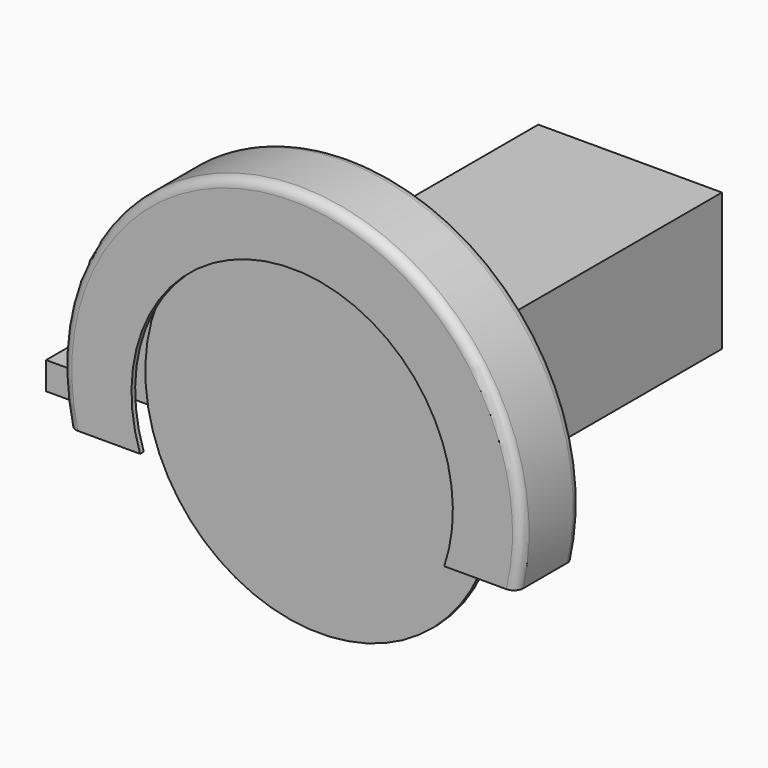
from build123d import *

# Parameters (mm, degrees)
F1_DEPTH  = 20
F2_T      = -2.5
F3_START  = -17.5
F3_DEPTH  = 2.5
F4_START  = -17.5
F0_W      = 100
F0_H      = 75
F4_DEPTH  = 192.5
F5_R      = 5
F6_DEPTH  = 1.2
F7_W      = 15
F7_H      = 15
F8_DEPTH  = 100
F9_W      = 15
F9_H      = 15
F10_DEPTH = 20


with BuildPart() as f1:
    # F0 (on Front) → F1 (new body, symmetric)
    with BuildSketch(Plane.XZ):
        with BuildLine():
            ThreePointArc((-93.7288880384, -32.7305903801), (-17.3139573127, 89.4389150959), (91.973567456, -4.4805537909))
            ThreePointArc((91.973567456, -4.4805537909), (90.8930363428, -18.7680785596), (87.6760229504, -32.7305903801))
            Line((87.6760229504, -32.7305903801), (118.739471685, -32.7305903801))
            ThreePointArc((118.739471685, -32.7305903801), (-3.026432544, 120.5194462091), (-124.792336773, -32.7305903801))
            Line((-124.792336773, -32.7305903801), (-93.7288880384, -32.7305903801))
        make_face()
        with BuildLine():
            ThreePointArc((87.6760229504, -32.7305903801), (90.8930363428, -18.7680785596), (91.973567456, -4.4805537909))
            ThreePointArc((91.973567456, -4.4805537909), (-17.3139573127, 89.4389150959), (-93.7288880384, -32.7305903801))
            Line((-93.7288880384, -32.7305903801), (-85.8405945739, -32.7305903801))
            ThreePointArc((-85.8405945739, -32.7305903801), (-3.026432544, 83.0194462091), (79.7877294859, -32.7305903801))
            Line((79.7877294859, -32.7305903801), (87.6760229504, -32.7305903801))
        make_face()
    extrude(amount=F1_DEPTH, both=True)

    # F2
    f2_openings = [f1.faces().sort_by_distance(p)[0] for p in [
        (-3.026433, 0, 83.019446),
        (99.263601, 0, -32.73059),
        (-105.316466, 0, -32.73059),
    ]]
    offset(amount=F2_T, openings=f2_openings)

    # F0 (on Front) → F3 (join)
    with BuildSketch(Plane.XZ.offset(F3_START)):
        with BuildLine():
            ThreePointArc((79.7877294859, -32.7305903801), (-3.026432544, 83.0194462091), (-85.8405945739, -32.7305903801))
            Line((-85.8405945739, -32.7305903801), (-53.026432544, -32.7305903801))
            Line((-53.026432544, -32.7305903801), (-53.026432544, 42.2694096199))
            Line((-53.026432544, 42.2694096199), (46.973567456, 42.2694096199))
            Line((46.973567456, 42.2694096199), (46.973567456, -32.7305903801))
            Line((46.973567456, -32.7305903801), (79.7877294859, -32.7305903801))
        make_face()
    extrude(amount=-F3_DEPTH)

    # F0 (on Front) → F4 (join)
    with BuildSketch(Plane.XZ.offset(F4_START)):
        with Locations((-3.026432544, 4.7694096199)):
            Rectangle(F0_W, F0_H)
    extrude(amount=-F4_DEPTH)

    # F5
    f5_edges = [f1.edges().sort_by_distance(p)[0] for p in [
        (-3.026433, -20, 120.519446),
        (-3.026433, 20, 120.519446),
    ]]
    fillet(f5_edges, radius=F5_R)

    # F7 (on face) → F8 (join)
    with BuildSketch(Plane(origin=(-53.026432544, 0, 0), x_dir=(0, -1, 0), z_dir=(-1, 0, 0))):
        with Locations((-27.5, -25.2305903801)):
            Rectangle(F7_W, F7_H)
    extrude(amount=F8_DEPTH)


with BuildPart() as f6:
    # F0 (on Front) → F6 (new body, symmetric)
    with BuildSketch(Plane.XZ):
        with BuildLine():
            ThreePointArc((87.6760229504, -32.7305903801), (90.8930363428, -18.7680785596), (91.973567456, -4.4805537909))
            ThreePointArc((91.973567456, -4.4805537909), (-17.3139573127, 89.4389150959), (-93.7288880384, -32.7305903801))
            Line((-93.7288880384, -32.7305903801), (-85.8405945739, -32.7305903801))
            ThreePointArc((-85.8405945739, -32.7305903801), (-3.026432544, 83.0194462091), (79.7877294859, -32.7305903801))
            Line((79.7877294859, -32.7305903801), (87.6760229504, -32.7305903801))
        make_face()
        with BuildLine():
            ThreePointArc((79.7877294859, -32.7305903801), (-3.026432544, 83.0194462091), (-85.8405945739, -32.7305903801))
            Line((-85.8405945739, -32.7305903801), (-53.026432544, -32.7305903801))
            Line((-53.026432544, -32.7305903801), (-53.026432544, 42.2694096199))
            Line((-53.026432544, 42.2694096199), (46.973567456, 42.2694096199))
            Line((46.973567456, 42.2694096199), (46.973567456, -32.7305903801))
            Line((46.973567456, -32.7305903801), (79.7877294859, -32.7305903801))
        make_face()
        with Locations((-3.026432544, 4.7694096199)):
            Rectangle(F0_W, F0_H)
        with BuildLine():
            Line((-85.8405945739, -32.7305903801), (-93.7288880384, -32.7305903801))
            ThreePointArc((-93.7288880384, -32.7305903801), (-3.026432544, -99.4805537909), (87.6760229504, -32.7305903801))
            Line((87.6760229504, -32.7305903801), (79.7877294859, -32.7305903801))
            Line((79.7877294859, -32.7305903801), (46.973567456, -32.7305903801))
            Line((46.973567456, -32.7305903801), (-53.026432544, -32.7305903801))
            Line((-53.026432544, -32.7305903801), (-85.8405945739, -32.7305903801))
        make_face()
    extrude(amount=F6_DEPTH, both=True)


with BuildPart() as f10:
    # F9 (on face) → F10 (new body)
    with BuildSketch(Plane.XZ.offset(-20)):
        with Locations((-145.526432544, -25.2305903801)):
            Rectangle(F9_W, F9_H)
    extrude(amount=F10_DEPTH)


solid = Compound([f1.part, f6.part, f10.part])
